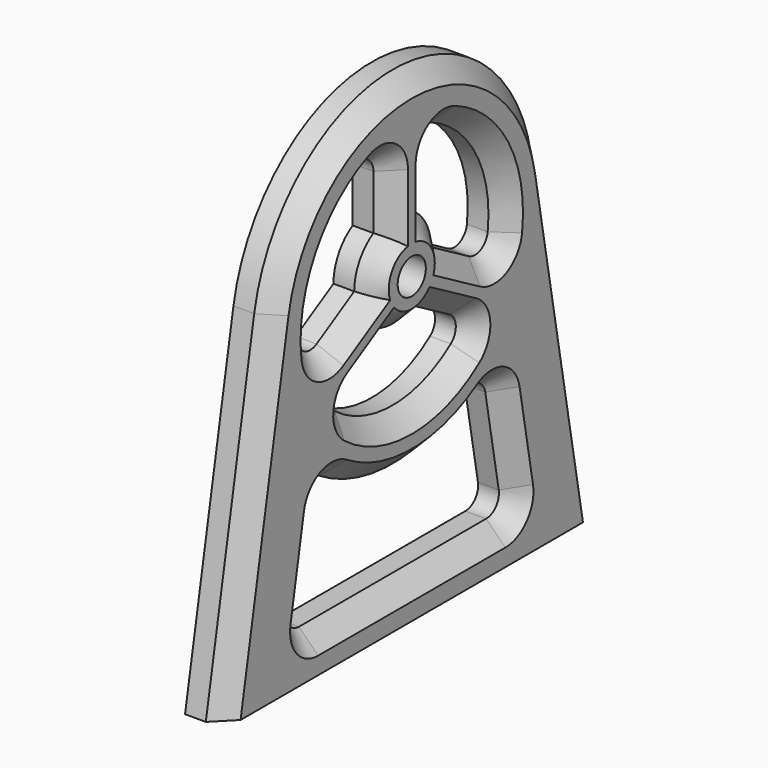
from build123d import *

# Parameters (mm, degrees)
F0_R     = 11
F1_DEPTH = 12.5
F2_SIZE  = 12
F3_R     = 10
F4_SIZE  = 12


# Not quite as in the source:
# - a feature names something its author has since deleted; it is built from what else it names


with BuildPart() as f1:
    # F0 (on Right) → F1 (new body, symmetric)
    with BuildSketch(Plane.YZ):
        with BuildLine():
            Line((-108.2477509669, 143.9956215311), (-146.1053743867, -65.5600531085))
            Line((-146.1053743867, -65.5600531085), (0, -65.5600531085))
            Line((0, -65.5600531085), (146.1053743867, -65.5600531085))
            Line((146.1053743867, -65.5600531085), (108.2477509669, 143.9956215311))
            ThreePointArc((108.2477509669, 143.9956215311), (0, 234.4399468915), (-108.2477509669, 143.9956215311))
        make_face()
        with BuildLine():
            Line((-85.1559906377, -42.7505690663), (-69.6519457463, 43.0699419263))
            ThreePointArc((-69.6519457463, 43.0699419263), (0, 17.3303242879), (69.6519457463, 43.0699419263))
            Line((69.6519457463, 43.0699419263), (85.1559906377, -42.7505690663))
            Line((85.1559906377, -42.7505690663), (0, -42.7505690663))
            Line((0, -42.7505690663), (-85.1559906377, -42.7505690663))
        make_face(mode=Mode.SUBTRACT)
        with BuildLine():
            ThreePointArc((56.1396103068, 74.707219693), (0, 49.4399468915), (-56.1396103068, 74.707219693))
            Line((-56.1396103068, 74.707219693), (-15, 98.459184778))
            ThreePointArc((-15, 98.459184778), (0, 94.4399468915), (15, 98.459184778))
            Line((15, 98.459184778), (56.1396103068, 74.707219693))
        make_face(mode=Mode.SUBTRACT)
        with BuildLine():
            Line((-15, 197.924639175), (-15, 150.420709005))
            ThreePointArc((-15, 150.420709005), (-25.9807621135, 139.4399468915), (-30, 124.4399468915))
            Line((-30, 124.4399468915), (-71.1396103068, 100.6879818065))
            ThreePointArc((-71.1396103068, 100.6879818065), (-64.9519052838, 161.9399468915), (-15, 197.924639175))
        make_face(mode=Mode.SUBTRACT)
        with Locations((0, 124.4399468915)):
            Circle(F0_R, mode=Mode.SUBTRACT)
        with BuildLine():
            Line((15, 150.420709005), (15, 197.924639175))
            ThreePointArc((15, 197.924639175), (64.9519052838, 161.9399468915), (71.1396103068, 100.6879818065))
            Line((71.1396103068, 100.6879818065), (30, 124.4399468915))
            ThreePointArc((30, 124.4399468915), (25.9807621135, 139.4399468915), (15, 150.420709005))
        make_face(mode=Mode.SUBTRACT)
    extrude(amount=F1_DEPTH, both=True)

    # F2
    f2_edges = [f1.edges().sort_by_distance(p)[0] for p in [
        (12.5, 0, 234.439947),
    ]]
    chamfer(f2_edges, length=F2_SIZE)

    # F3
    f3_edges = [f1.edges().sort_by_distance(p)[0] for p in [
        (0, -69.651946, 43.069942),
        (0, 69.651946, 43.069942),
        (0, -85.155991, -42.750569),
        (0, 85.155991, -42.750569),
        (0, -15, 197.924639),
        (0, 15, 197.924639),
        (0, -71.13961, 100.687982),
        (0, -56.13961, 74.70722),
        (0, 56.13961, 74.70722),
        (0, 71.13961, 100.687982),
    ]]
    fillet(f3_edges, radius=F3_R)

    # F4
    f4_edges = [f1.edges().sort_by_distance(p)[0] for p in [
        (12.5, 0, 17.330324),
        (12.5, -64.951905, 161.939947),
        (12.5, 64.951905, 161.939947),
        (12.5, 0, 49.439947),
        (12.5, -25.980762, 139.439947),
        (12.5, 0, 94.439947),
        (12.5, 25.980762, 139.439947),
    ]]
    chamfer(f4_edges, length=F4_SIZE)


solid = f1.part
